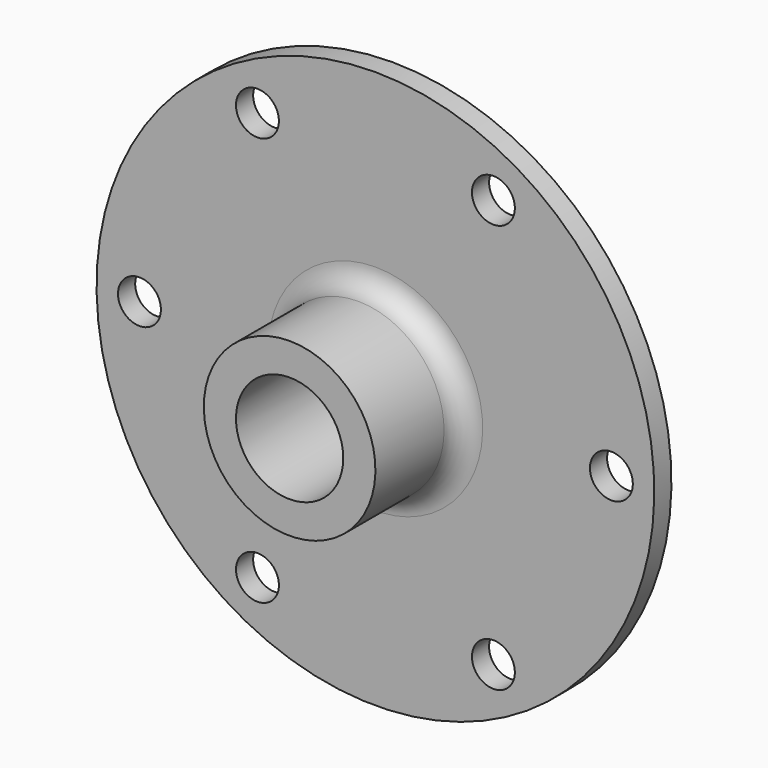
from build123d import *

# Parameters (mm, degrees)
F2_R            = 7.9375
F3_DEPTH        = 19.05
F4_R            = 3.175
F5_DEPTH        = 3.175
F5_COPIES_COUNT = 6
F6_R            = 3.175


# Not quite as in the source:
# - a pattern or mirror of a feature is missing from the dataset's text; its kind, count and spacing are read off the source's solid


with BuildPart() as f1:
    # F0 (on Right) → F1 (revolve)
    with BuildSketch(Plane.YZ):
        Polygon((0, 0), (0, 41.275), (-3.175, 41.275), (-3.175, 12.7), (-19.05, 12.7), (-19.05, 0), align=None)
    revolve(axis=Axis((0, -9.525, 0), (0, -1, 0)))

    # F2 (on face) → F3 (cut, through all)
    with BuildSketch(Plane.XZ.offset(19.05)):
        Circle(F2_R)
    extrude(amount=-F3_DEPTH, mode=Mode.SUBTRACT)

    # F4 (on face) → F5 (cut, through all)
    with BuildSketch(Plane.XZ.offset(3.175)):
        with Locations((34.925, 0)):
            Circle(F4_R)
    f5 = extrude(amount=-F5_DEPTH, mode=Mode.SUBTRACT)

    # F5_copies: F5 ×6 about axis
    f5_copies_axis = Axis((0, 0, 0), (0, 1, 0))
    for i in range(1, F5_COPIES_COUNT):
        add(f5.rotate(f5_copies_axis, i * 360 / F5_COPIES_COUNT), mode=Mode.SUBTRACT)

    # F6
    f6_edges = [f1.edges().sort_by_distance(p)[0] for p in [
        (0, -3.175, -12.7),
    ]]
    fillet(f6_edges, radius=F6_R)


solid = f1.part
